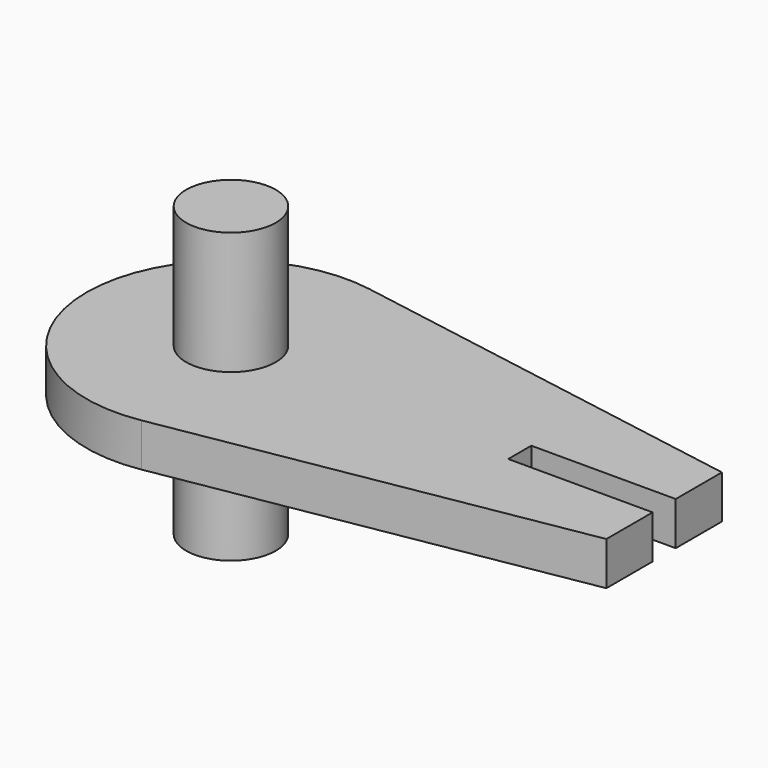
from build123d import *

# Parameters (mm, degrees)
F0_R     = 3.1
F1_DEPTH = 10
F2_DEPTH = 1.5
F3_W     = 10
F3_H     = 2
F4_DEPTH = 11.501


# Not quite as in the source:
# - a feature names something its author has since deleted; it is built from what else it names


with BuildPart() as f1:
    # F0 (on Top) → F1 (new body, symmetric)
    with BuildSketch(Plane.XY):
        Circle(F0_R)
    extrude(amount=F1_DEPTH, both=True)

    # F0 (on Top) → F2 (join, symmetric)
    with BuildSketch(Plane.XY):
        with BuildLine():
            ThreePointArc((1.6906574466, -9.8560477575), (7.6454749514, -6.4456739576), (10, 0))
            ThreePointArc((10, 0), (7.6454749525, 6.4456739563), (1.6906574499, 9.8560477569))
            ThreePointArc((1.6906574499, 9.8560477569), (-10, 1.7e-09), (1.6906574466, -9.8560477575))
        make_face()
        Circle(F0_R, mode=Mode.SUBTRACT)
        with BuildLine():
            ThreePointArc((1.6906574499, 9.8560477569), (7.6454749525, 6.4456739563), (10, 0))
            ThreePointArc((10, 0), (7.6454749514, -6.4456739576), (1.6906574466, -9.8560477575))
            Line((1.6906574466, -9.8560477575), (30, -5))
            Line((30, -5), (30, 5))
            Line((30, 5), (1.6906574499, 9.8560477569))
        make_face()
    extrude(amount=F2_DEPTH, both=True)

    # F3 (on face) → F4 (cut, through all)
    with BuildSketch(Plane.XY.offset(1.5)):
        with Locations((25, 0)):
            Rectangle(F3_W, F3_H)
    extrude(amount=-F4_DEPTH, mode=Mode.SUBTRACT)


solid = f1.part
